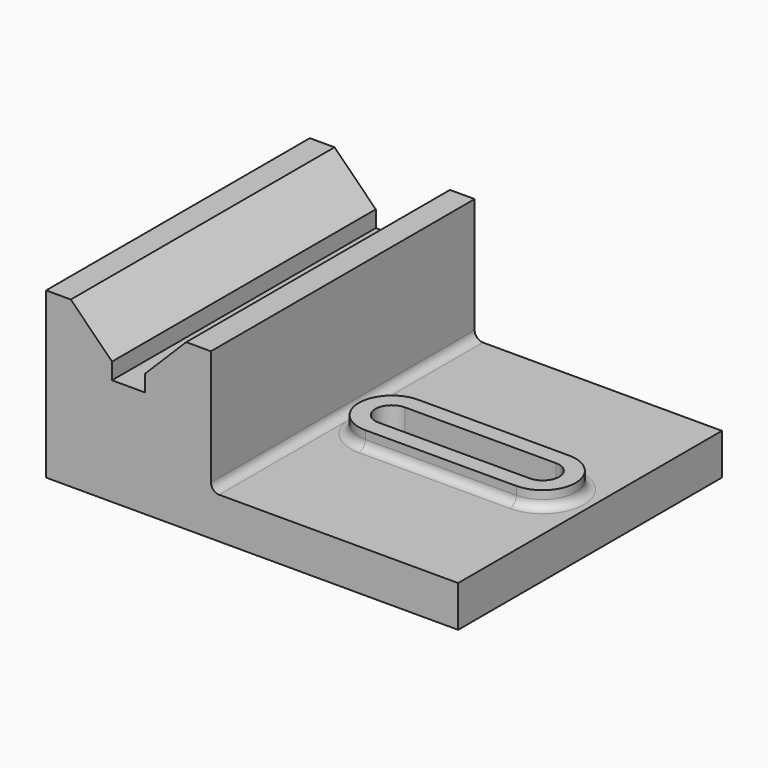
from build123d import *

# Parameters (mm, degrees)
F1_DEPTH    = 200
F3_DEPTH    = 10
F4_DEPTH    = 25
F5_T1_DEPTH = 200
F5_T3_DEPTH = 91.5131680667
F5_T6_ANGLE = 180
F5_T8_ANGLE = 180


# Not quite as in the source:
# - a fillet or chamfer that OpenCascade refuses, or shapes differently, is made with other operations: its cross-section is extruded or revolved along the edge and cut away or added


with BuildPart() as f1:
    # F0 (on Front) → F1 (new body)
    with BuildSketch(Plane.XZ):
        Polygon((-250, 0), (0, 0), (0, 25), (-150, 25), (-150, 100), (-165, 100), (-190, 75), (-190, 65), (-210, 65), (-210, 75), (-235, 100), (-250, 100), align=None)
    extrude(amount=F1_DEPTH)

    # F2 (on face) → F3 (join)
    with BuildSketch(Plane.XY.offset(25)):
        with BuildLine():
            Line((-120.2453300357, -120), (-28.7321619689, -120))
            ThreePointArc((-28.7321619689, -120), (-8.7321619689, -100), (-28.7321619689, -80))
            Line((-28.7321619689, -80), (-120.2453300357, -80))
            ThreePointArc((-120.2453300357, -80), (-140.2453300357, -100), (-120.2453300357, -120))
        make_face()
        with BuildLine():
            ThreePointArc((-28.7321619689, -90), (-18.7321619689, -100), (-28.7321619689, -110))
            Line((-28.7321619689, -110), (-120.2453300357, -110))
            ThreePointArc((-120.2453300357, -110), (-130.2453300357, -100), (-120.2453300357, -90))
            Line((-120.2453300357, -90), (-28.7321619689, -90))
        make_face(mode=Mode.SUBTRACT)
    extrude(amount=F3_DEPTH)

    # F4 (cut): a face of the model
    f4_faces = [f1.faces().sort_by_distance(p)[0] for p in [
        (-74.4887460023, -100, 25),
    ]]
    extrude(f4_faces, amount=-F4_DEPTH, mode=Mode.SUBTRACT)

    # F5: fillet of radius 5 on 3 edges, made by hand

    # F5_s2 → F5_t1 (join)
    with BuildSketch(Plane.XZ):
        with BuildLine():
            ThreePointArc((-145, 25), (-148.5355339059, 26.4644660941), (-150, 30))
            Line((-150, 30), (-150, 25))
            Line((-150, 25), (-145, 25))
        make_face()
    extrude(amount=F5_T1_DEPTH)

    # F5_s4 → F5_t3 (join)
    with BuildSketch(Plane.YZ.offset(-120.2453300357)):
        with BuildLine():
            ThreePointArc((-125, 25), (-121.4644660941, 26.4644660941), (-120, 30))
            Line((-120, 30), (-120, 25))
            Line((-120, 25), (-125, 25))
        make_face()
        with BuildLine():
            ThreePointArc((-75, 25), (-78.5355339059, 26.4644660941), (-80, 30))
            Line((-80, 30), (-80, 25))
            Line((-80, 25), (-75, 25))
        make_face()
    extrude(amount=F5_T3_DEPTH)

    # F5_s5 → F5_t6 (revolve)
    with BuildSketch(Plane.YZ.offset(-28.7321619689)):
        with BuildLine():
            ThreePointArc((-120, 30), (-121.4644660941, 26.4644660941), (-125, 25))
            Line((-125, 25), (-120, 25))
            Line((-120, 25), (-120, 30))
        make_face()
    revolve(axis=Axis((-28.7321619689, -100, 25), (0, 0, 1)), revolution_arc=F5_T6_ANGLE)

    # F5_s7 → F5_t8 (revolve)
    with BuildSketch(Plane.YZ.offset(-120.2453300357)):
        with BuildLine():
            ThreePointArc((-75, 25), (-78.5355339059, 26.4644660941), (-80, 30))
            Line((-80, 30), (-80, 25))
            Line((-80, 25), (-75, 25))
        make_face()
    revolve(axis=Axis((-120.2453300357, -100, 25), (0, 0, 1)), revolution_arc=F5_T8_ANGLE)


solid = f1.part
